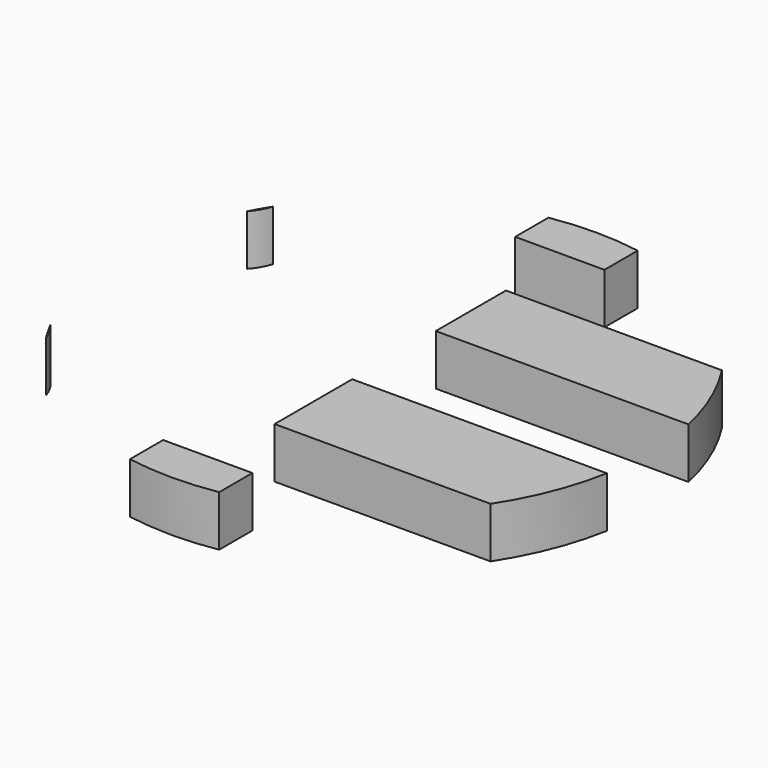
from build123d import *

# Parameters (mm, degrees)
F1_DEPTH = 5


# Not quite as in the source:
# - a feature names something its author has since deleted; it is built from what else it names


with BuildPart() as f1:
    # F0 (on Top) → F1 (new body)
    with BuildSketch(Plane.XY):
        with BuildLine():
            Line((-10.0905321275, 5.8453546624), (14.8275429309, 5.8453546624))
            ThreePointArc((14.8275429309, 5.8453546624), (13.4089467522, 10.333836128), (11.2090090081, 14.4954650047))
            Line((11.2090090081, 14.4954650047), (-10.0905321275, 14.4954650047))
            Line((-10.0905321275, 14.4954650047), (-10.0905321275, 5.8453546624))
        make_face()
    extrude(amount=F1_DEPTH)


with BuildPart() as f1b:
    # F0 (on Top) → F1, piece 2 (new body)
    with BuildSketch(Plane.XY):
        with BuildLine():
            Line((-10.0905321275, -14.0213307756), (11.2090090081, -14.0213307756))
            ThreePointArc((11.2090090081, -14.0213307756), (13.5867060203, -9.4237936022), (15.0127789753, -4.4481421807))
            Line((15.0127789753, -4.4481421807), (-10.0905321275, -4.4481421807))
            Line((-10.0905321275, -4.4481421807), (-10.0905321275, -14.0213307756))
        make_face()
    extrude(amount=F1_DEPTH)


with BuildPart() as f1c:
    # F0 (on Top) → F1, piece 3 (new body)
    with BuildSketch(Plane.XY):
        with BuildLine():
            Line((-15.1280330338, -21.4612806617), (-15.1280330338, -25.5532806617))
            ThreePointArc((-15.1280330338, -25.5532806617), (-10.7273935254, -25.9260303035), (-6.326754017, -25.5532806617))
            Line((-6.326754017, -25.5532806617), (-6.326754017, -21.4612806617))
            Line((-6.326754017, -21.4612806617), (-15.1280330338, -21.4612806617))
        make_face()
    extrude(amount=F1_DEPTH)


with BuildPart() as f1d:
    # F0 (on Top) → F1, piece 4 (new body)
    with BuildSketch(Plane.XY):
        with BuildLine():
            ThreePointArc((-32.8259622054, -13.7686791634), (-33.2689093484, -12.7551765215), (-33.9238437811, -11.8638569014))
            ThreePointArc((-33.9238437811, -11.8638569014), (-33.3949203437, -12.8278054239), (-32.8259622054, -13.7686791634))
        make_face()
    extrude(amount=F1_DEPTH)


with BuildPart() as f1e:
    # F0 (on Top) → F1, piece 5 (new body)
    with BuildSketch(Plane.XY):
        with BuildLine():
            ThreePointArc((-33.907864258, 12.3685733327), (-33.2698270825, 13.2408768133), (-32.8341372879, 14.2299062378))
            ThreePointArc((-32.8341372879, 14.2299062378), (-33.3901181901, 13.3102678428), (-33.907864258, 12.3685733327))
        make_face()
    extrude(amount=F1_DEPTH)


with BuildPart() as f1f:
    # F0 (on Top) → F1, piece 6 (new body)
    with BuildSketch(Plane.XY):
        with BuildLine():
            Line((-6.326754017, 21.931238229), (-6.326754017, 26.0274148909))
            ThreePointArc((-6.326754017, 26.0274148909), (-10.7273935254, 26.4001645326), (-15.1280330338, 26.0274148909))
            Line((-15.1280330338, 26.0274148909), (-15.1280330338, 21.931238229))
            Line((-15.1280330338, 21.931238229), (-6.326754017, 21.931238229))
        make_face()
    extrude(amount=F1_DEPTH)


solid = Compound([f1.part, f1b.part, f1c.part, f1d.part, f1e.part, f1f.part])
